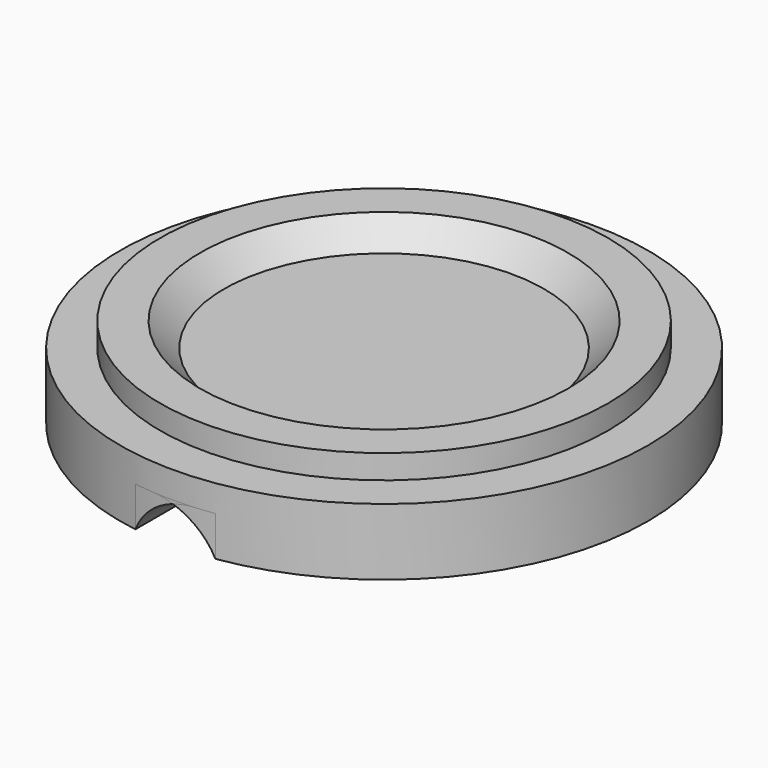
from build123d import *

# Parameters (mm, degrees)
F0_R         = 19.8
F1_DEPTH     = 5
F2_R         = 16.8
F2_R_2       = 16
F3_DEPTH     = 1.8
F6_DEPTH     = 3
F7_T4_DEPTH  = 62.0556939075
F7_S5_R      = 19.8
F7_T6_DEPTH  = 33
F7_T10_DEPTH = 62.0556939075
F7_S11_R     = 19.8
F7_T12_DEPTH = 33


# Not quite as in the source:
# - a fillet or chamfer that OpenCascade refuses, or shapes differently, is made with other operations: its cross-section is extruded or revolved along the edge and cut away or added


with BuildPart() as f1:
    # F0 (on Top) → F1 (new body)
    with BuildSketch(Plane.XY):
        Circle(F0_R)
    extrude(amount=F1_DEPTH)

    # F2 (on face) → F3 (join)
    with BuildSketch(Plane.XY.offset(5)):
        Circle(F2_R)
        Circle(F2_R_2, mode=Mode.SUBTRACT)
    extrude(amount=F3_DEPTH)

    # F4: chamfer of 4 on 1 edges, made by hand


with BuildPart() as f4_tool2:
    # F4_s3 → F4_t4 (revolve)
    with BuildSketch(Plane.XZ):
        Polygon((16, 9), (12, 5), (16, 5), align=None)
    revolve(axis=Axis((0, 0, 5), (0, 0, 1)))

    split(bisect_by=Plane.XY.offset(6.8), keep=Keep.BOTTOM)


with BuildPart() as f1_1:
    add(f1.part)

    # F4_t1: union F4_tool2
    add(f4_tool2.part)

    # F5 (on face) → F6 (cut)
    with BuildSketch(Plane(origin=(0, 0, 0), x_dir=(1, 0, 0), z_dir=(0, 0, -1))):
        with BuildLine():
            Line((-3, 19.5714077164), (-3, -19.5714077164))
            ThreePointArc((-3, -19.5714077164), (0, -19.8), (3, -19.5714077164))
            Line((3, -19.5714077164), (3, 19.5714077164))
            ThreePointArc((3, 19.5714077164), (0, 19.8), (-3, 19.5714077164))
        make_face()
    extrude(amount=-F6_DEPTH, mode=Mode.SUBTRACT)

    # F7: fillet of radius 5 on 2 edges, made by hand


with BuildPart() as f7_tool2:
    # F7_s3 → F7_t4 (new body)
    with BuildSketch(Plane.XZ.offset(-31.0278469537)):
        with BuildLine():
            ThreePointArc((3, 0), (1.1560370926, 2.1833001327), (-1.582575695, 3))
            Line((-1.582575695, 3), (3, 3))
            Line((3, 3), (3, 0))
        make_face()
    extrude(amount=F7_T4_DEPTH)

    # F7_s5 → F7_t6 (intersect, symmetric)
    with BuildSketch(Plane.XY.offset(1.5)):
        Circle(F7_S5_R)
    extrude(amount=F7_T6_DEPTH, both=True, mode=Mode.INTERSECT)


with BuildPart() as f1_2:
    add(f1_1.part)

    # F7_t1: union F7_tool2
    add(f7_tool2.part)


with BuildPart() as f7_tool8:
    # F7_s9 → F7_t10 (new body)
    with BuildSketch(Plane.XZ.offset(31.0278469537)):
        with BuildLine():
            ThreePointArc((1.582575695, 3), (-1.1560370926, 2.1833001327), (-3, 0))
            Line((-3, 0), (-3, 3))
            Line((-3, 3), (1.582575695, 3))
        make_face()
    extrude(amount=-F7_T10_DEPTH)

    # F7_s11 → F7_t12 (intersect, symmetric)
    with BuildSketch(Plane.XY.offset(1.5)):
        Circle(F7_S11_R)
    extrude(amount=F7_T12_DEPTH, both=True, mode=Mode.INTERSECT)


with BuildPart() as f1_3:
    add(f1_2.part)

    # F7_t7: union F7_tool8
    add(f7_tool8.part)


solid = f1_3.part
